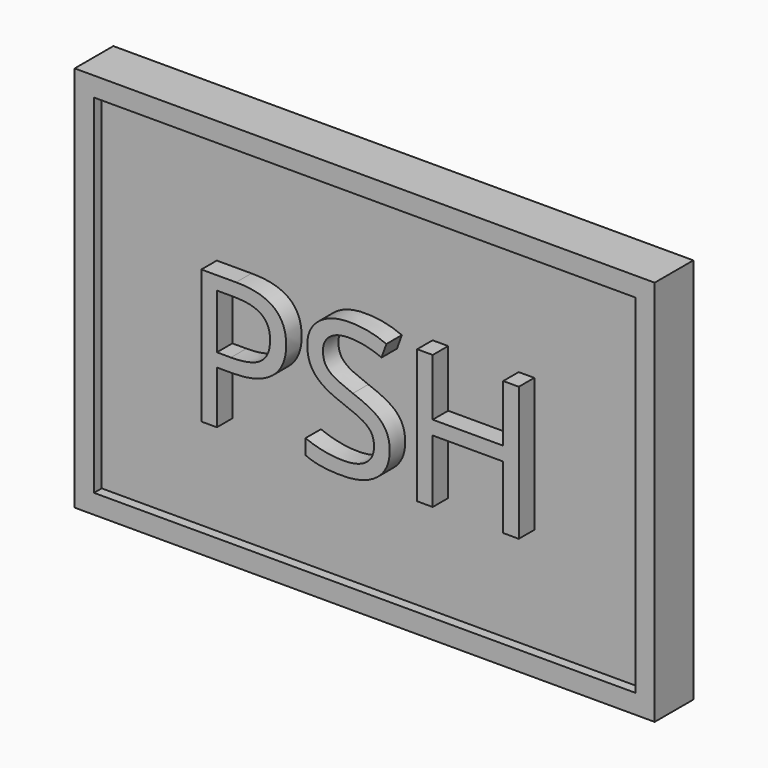
from build123d import *

# Parameters (mm, degrees)
F0_W         = 300
F0_H         = 200
F1_DEPTH     = 25
F2_W         = 280
F2_H         = 180
F3_DEPTH     = 5
F4_W         = 150
F4_H         = 100
F5_DEPTH     = 20
F6_R         = 10
F7_DEPTH     = 15
F8_TEXT_SIZE = 96.9860245833
F9_DEPTH     = 10


# Not quite as in the source:
# - Text() gives the source's letters only with a copy of the font that has no kerning and outlines rounded to 1/6400 em; it was checked with that copy


with BuildPart() as f1:
    # F0 (on Front) → F1 (new body)
    with BuildSketch(Plane.XZ):
        Rectangle(F0_W, F0_H)
    extrude(amount=F1_DEPTH)

    # F2 (on face) → F3 (cut)
    with BuildSketch(Plane.XZ.offset(25)):
        Rectangle(F2_W, F2_H)
    extrude(amount=-F3_DEPTH, mode=Mode.SUBTRACT)

    # F4 (on face) → F5 (join)
    with BuildSketch(Plane(origin=(0, 0, 0), x_dir=(-1, 0, 0), z_dir=(0, 1, 0))):
        Rectangle(F4_W, F4_H)
    extrude(amount=F5_DEPTH)

    # F6 (on face) → F7 (join)
    with BuildSketch(Plane(origin=(0, 20, 0), x_dir=(-1, 0, 0), z_dir=(0, 1, 0))):
        Circle(F6_R)
    extrude(amount=F7_DEPTH)

    # F8 (on face) → F9 (join)
    with BuildSketch(Plane.XZ.offset(20)):
        with Locations((-90, -36.1561623562)):
            Text('PSH', F8_TEXT_SIZE, font='Open Sans', text_align=(TextAlign.LEFT, TextAlign.BOTTOM))
    extrude(amount=F9_DEPTH)


solid = f1.part
